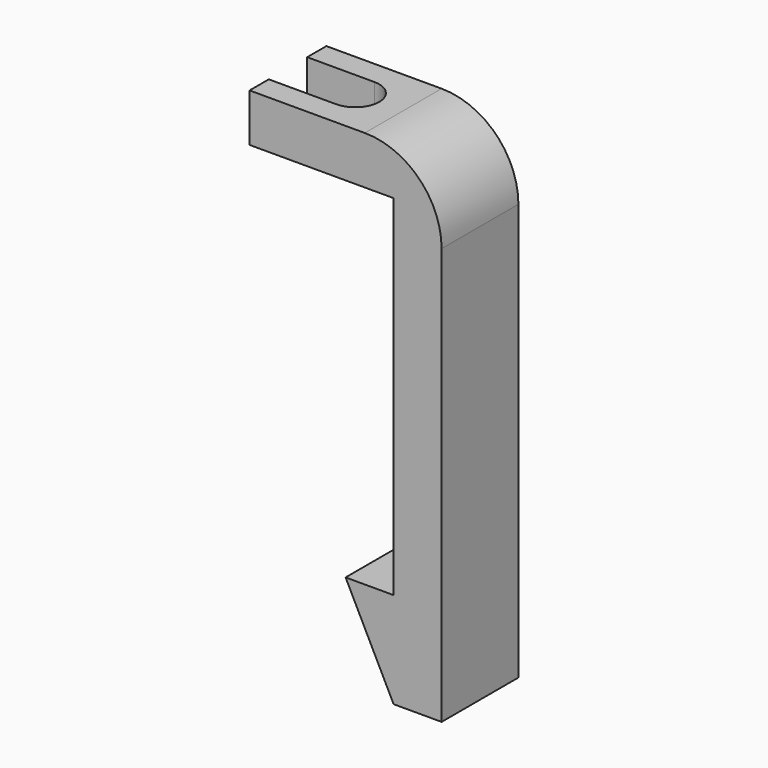
from build123d import *

# Parameters (mm, degrees)
F1_DEPTH = 6.35
F2_R     = 5.08
F4_DEPTH = 25.4
F5_W     = 8.255
F5_H     = 6.35
F6_DEPTH = 4.99459


with BuildPart() as f1:
    # F0 (on Front) → F1 (new body)
    with BuildSketch(Plane.XZ):
        Polygon((0, 3.175), (0, 0), (17.78, 0), (20.955, 0), (20.955, 3.175), align=None)
        Polygon((20.955, 0), (17.78, 0), (17.78, -23.114), (17.78, -29.464), (20.955, -29.464), align=None)
        Polygon((17.78, -29.464), (17.78, -23.114), (14.605, -23.114), align=None)
    extrude(amount=F1_DEPTH)

    # F2
    f2_edges = [f1.edges().sort_by_distance(p)[0] for p in [
        (20.955, -3.175, 3.175),
    ]]
    fillet(f2_edges, radius=F2_R)

    # F3 (on face) → F4 (cut)
    with BuildSketch(Plane.XY.offset(3.175)):
        with BuildLine():
            ThreePointArc((4.1275, -3.175), (3.6625320151, -4.2975320151), (2.54, -4.7625))
            Line((2.54, -4.7625), (12.7, -4.7625))
            ThreePointArc((12.7, -4.7625), (11.1125, -3.175), (12.7, -1.5875))
            Line((12.7, -1.5875), (2.54, -1.5875))
            ThreePointArc((2.54, -1.5875), (3.6625320151, -2.0524679849), (4.1275, -3.175))
        make_face()
        with BuildLine():
            ThreePointArc((2.54, -1.5875), (0.9525, -3.175), (2.54, -4.7625))
            Line((2.54, -4.7625), (2.54, -1.5875))
        make_face()
        with BuildLine():
            Line((2.54, -1.5875), (2.54, -4.7625))
            ThreePointArc((2.54, -4.7625), (3.6625320151, -4.2975320151), (4.1275, -3.175))
            ThreePointArc((4.1275, -3.175), (3.6625320151, -2.0524679849), (2.54, -1.5875))
        make_face()
        with BuildLine():
            ThreePointArc((12.7, -1.5875), (11.1125, -3.175), (12.7, -4.7625))
            Line((12.7, -4.7625), (12.7, -1.5875))
        make_face()
        with BuildLine():
            Line((12.7, -1.5875), (12.7, -4.7625))
            ThreePointArc((12.7, -4.7625), (13.8225320151, -4.2975320151), (14.2875, -3.175))
            ThreePointArc((14.2875, -3.175), (13.8225320151, -2.0524679849), (12.7, -1.5875))
        make_face()
    extrude(amount=-F4_DEPTH, mode=Mode.SUBTRACT)

    # F5 (on face) → F6 (cut)
    with BuildSketch(Plane.XY.offset(3.175)):
        with Locations((4.1275, -3.175)):
            Rectangle(F5_W, F5_H)
    extrude(amount=-F6_DEPTH, mode=Mode.SUBTRACT)


solid = f1.part
